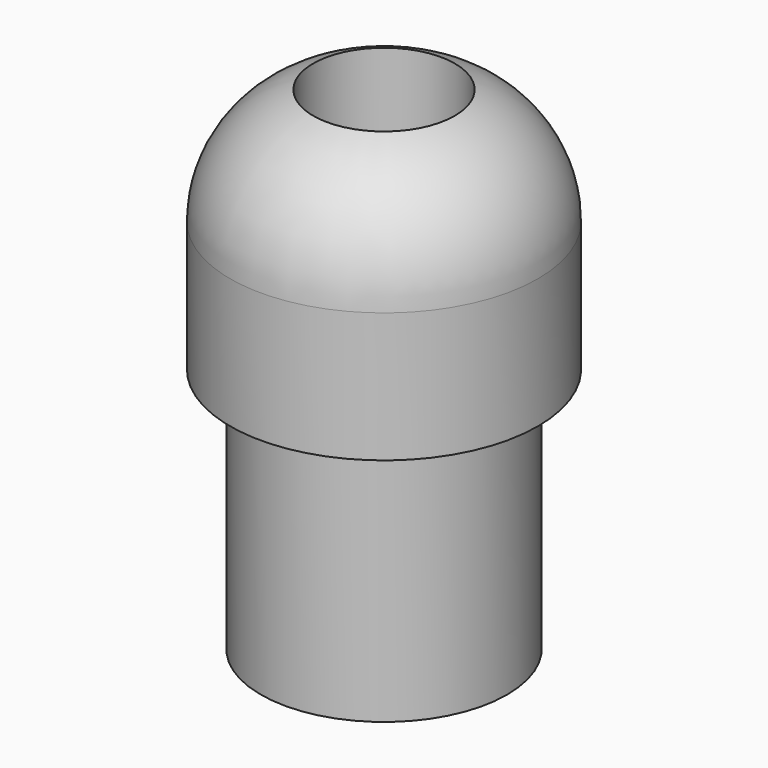
from build123d import *

# Parameters (mm, degrees)
F0_R     = 2
F0_R_2   = 1.15
F1_DEPTH = 8
F3_R     = 2.5
F3_R_2   = 2
F4_DEPTH = 4


# Not quite as in the source:
# - a fillet or chamfer that OpenCascade refuses, or shapes differently, is made with other operations: its cross-section is extruded or revolved along the edge and cut away or added


with BuildPart() as f1:
    # F0 (on Top) → F1 (new body)
    with BuildSketch(Plane.XY):
        Circle(F0_R)
        Circle(F0_R_2, mode=Mode.SUBTRACT)
    extrude(amount=F1_DEPTH)

    # F3 (on offset) → F4 (join, through all)
    with BuildSketch(Plane.XY.offset(4)):
        Circle(F3_R)
        Circle(F3_R_2, mode=Mode.SUBTRACT)
    extrude(amount=F4_DEPTH)

    # F5: fillet of radius 2 on 1 edges, made by hand

    # F5_s1 → F5_t2 (revolve, cut)
    with BuildSketch(Plane.XZ):
        with BuildLine():
            ThreePointArc((2.5, 6.1085719681), (2.1278820596, 7.2704669719), (1.15, 8))
            Line((1.15, 8), (2.5, 8))
            Line((2.5, 8), (2.5, 6.1085719681))
        make_face()
    revolve(axis=Axis((0, 0, 8), (0, 0, 1)), mode=Mode.SUBTRACT)


solid = f1.part
